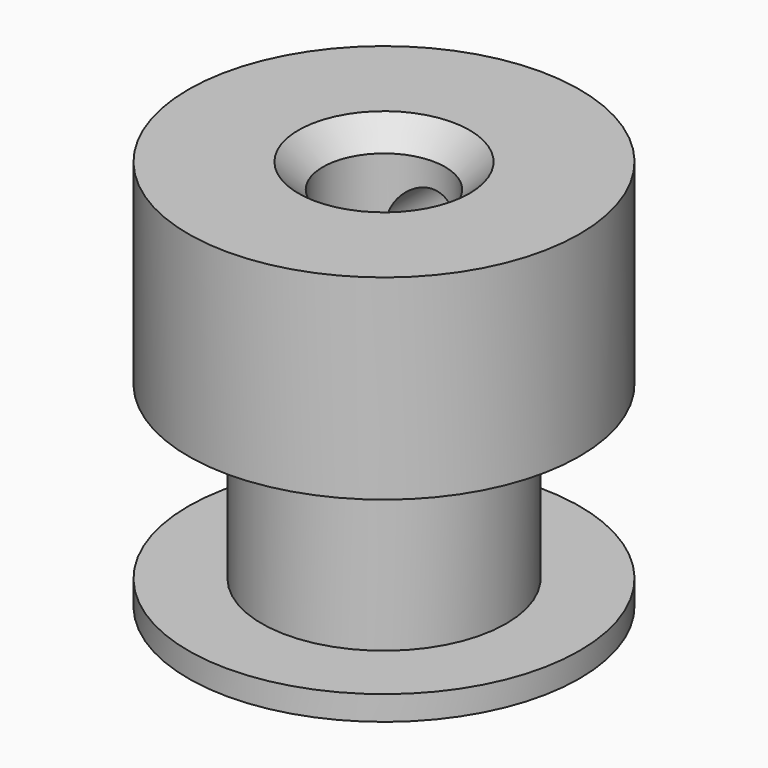
from build123d import *

# Parameters (mm, degrees)
F0_R     = 5
F0_R_2   = 2.5
F1_DEPTH = 3.5
F2_R     = 8
F2_R_2   = 2.5
F3_DEPTH = 1
F5_R     = 8
F5_R_2   = 2.5
F6_DEPTH = 7
F7_SIZE  = 1
F8_R     = 1.5
F9_DEPTH = 8.001


# Not quite as in the source:
# - a feature names something its author has since deleted; it is built from what else it names


with BuildPart() as f1:
    # F0 (on Top) → F1 (new body, symmetric)
    with BuildSketch(Plane.XY):
        Circle(F0_R)
        Circle(F0_R_2, mode=Mode.SUBTRACT)
    extrude(amount=F1_DEPTH, both=True)

    # F2 (on face) → F3 (join)
    with BuildSketch(Plane.XY.offset(3.5)):
        Circle(F2_R)
        Circle(F2_R_2, mode=Mode.SUBTRACT)
    extrude(amount=F3_DEPTH)

    # F4: F1 across plane


with BuildPart() as f1_1:
    add(f1.part)
    add(f1.part.mirror(Plane.XY))

    # F5 (on face) → F6 (join)
    with BuildSketch(Plane.XY.offset(4.5)):
        Circle(F5_R)
        Circle(F5_R_2, mode=Mode.SUBTRACT)
    extrude(amount=F6_DEPTH)

    # F7
    f7_edges = [f1_1.edges().sort_by_distance(p)[0] for p in [
        (-2.5, 0, 11.5),
        (-2.5, 0, -4.5),
    ]]
    chamfer(f7_edges, length=F7_SIZE)

    # F8 (on Front) → F9 (cut, through all)
    with BuildSketch(Plane.XZ):
        with Locations((0, 8)):
            Circle(F8_R)
    extrude(amount=-F9_DEPTH, mode=Mode.SUBTRACT)


solid = f1_1.part
